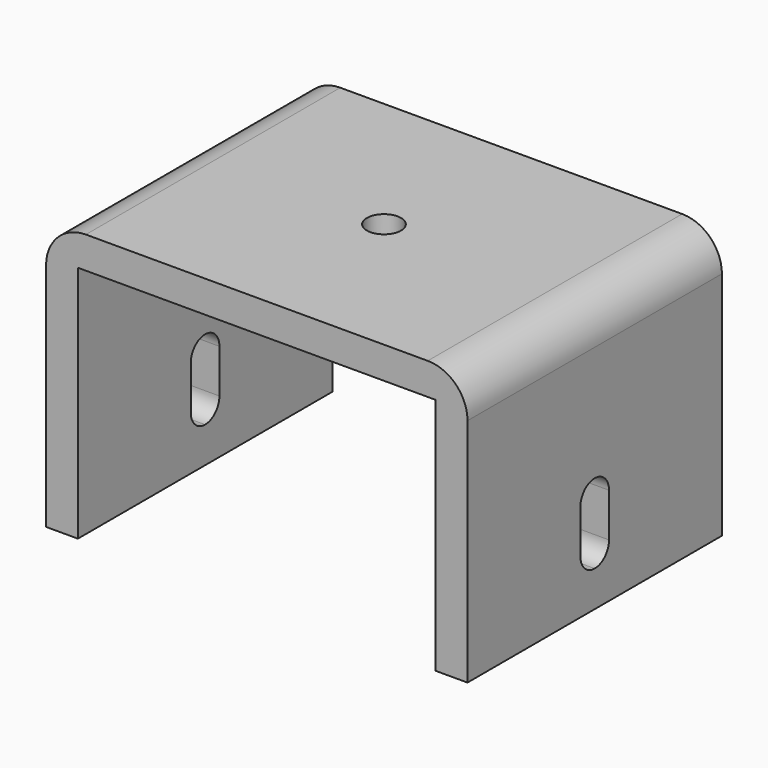
from build123d import *

# Parameters (mm, degrees)
F1_DEPTH = 40
F2_R     = 5
F3_R     = 2.15
F4_DEPTH = 25
F5_W     = 4.5
F5_H     = 10
F6_DEPTH = 53.001
F7_R     = 2.24999


# Not quite as in the source:
# - a fillet or chamfer is up to 0.001 mm smaller than in the source, because OpenCascade refuses the exact size


with BuildPart() as f1:
    # F0 (on Front) → F1 (new body)
    with BuildSketch(Plane.XZ):
        Polygon((22.5, -17), (26.5, -17), (26.5, 17), (-26.5, 17), (-26.5, -17), (-22.5, -17), (-22.5, 13), (22.5, 13), align=None)
    extrude(amount=F1_DEPTH)

    # F2
    f2_edges = [f1.edges().sort_by_distance(p)[0] for p in [
        (-26.5, -20, 17),
        (26.5, -20, 17),
    ]]
    fillet(f2_edges, radius=F2_R)

    # F3 (on face) → F4 (cut)
    with BuildSketch(Plane.XY.offset(17)):
        with Locations((0, -20)):
            Circle(F3_R)
    extrude(amount=-F4_DEPTH, mode=Mode.SUBTRACT)

    # F5 (on face) → F6 (cut, through all)
    with BuildSketch(Plane.YZ.offset(26.5)):
        with Locations((-20, -7.5)):
            Rectangle(F5_W, F5_H)
    extrude(amount=-F6_DEPTH, mode=Mode.SUBTRACT)

    # F7 (radius 2.25 in the source; OpenCascade refuses exactly that, so slightly less here)
    f7_edges = [f1.edges().sort_by_distance(p)[0] for p in [
        (24.5, -17.75, -2.5),
        (24.5, -22.25, -2.5),
        (24.5, -17.75, -12.5),
        (24.5, -22.25, -12.5),
        (-24.5, -17.75, -2.5),
        (-24.5, -17.75, -12.5),
        (-24.5, -22.25, -2.5),
        (-24.5, -22.25, -12.5),
    ]]
    fillet(f7_edges, radius=F7_R)


solid = f1.part
